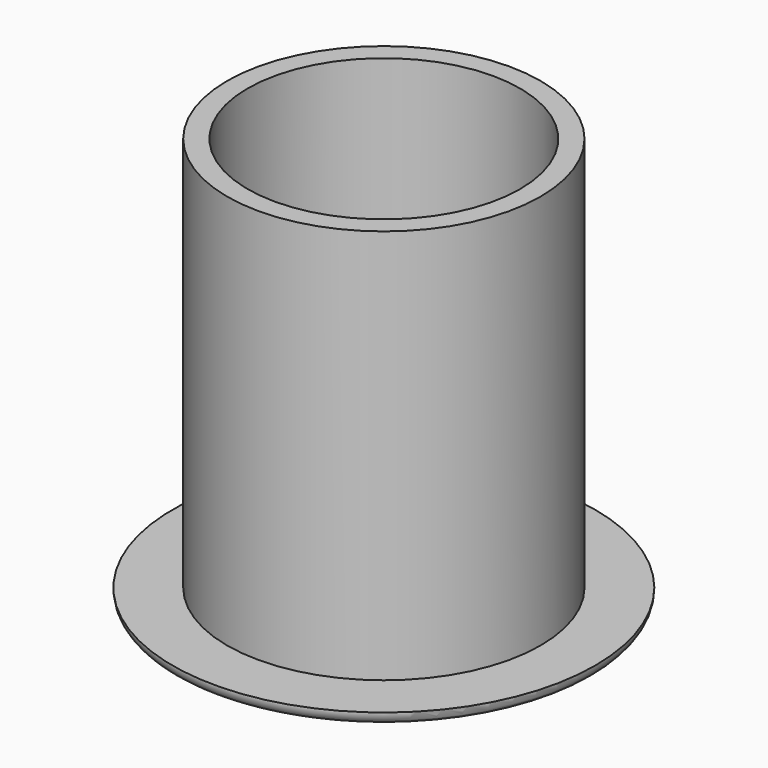
from build123d import *

# Parameters (mm, degrees)
F0_R     = 23
F0_R_2   = 20
F1_DEPTH = 60
F0_R_3   = 31
F2_DEPTH = 2
F3_R     = 1.99999
F4_R     = 5


# Not quite as in the source:
# - a fillet or chamfer is up to 0.001 mm smaller than in the source, because OpenCascade refuses the exact size


with BuildPart() as f1:
    # F0 (on Top) → F1 (new body)
    with BuildSketch(Plane.XY):
        Circle(F0_R)
        Circle(F0_R_2, mode=Mode.SUBTRACT)
    extrude(amount=F1_DEPTH)

    # F0 (on Top) → F2 (join)
    with BuildSketch(Plane.XY):
        Circle(F0_R_3)
        Circle(F0_R, mode=Mode.SUBTRACT)
    extrude(amount=F2_DEPTH)

    # F3 (radius 2 in the source; OpenCascade refuses exactly that, so slightly less here)
    f3_edges = [f1.edges().sort_by_distance(p)[0] for p in [
        (-31, 0, 0),
    ]]
    fillet(f3_edges, radius=F3_R)

    # F4
    f4_edges = [f1.edges().sort_by_distance(p)[0] for p in [
        (-20, 0, 0),
    ]]
    fillet(f4_edges, radius=F4_R)


solid = f1.part
